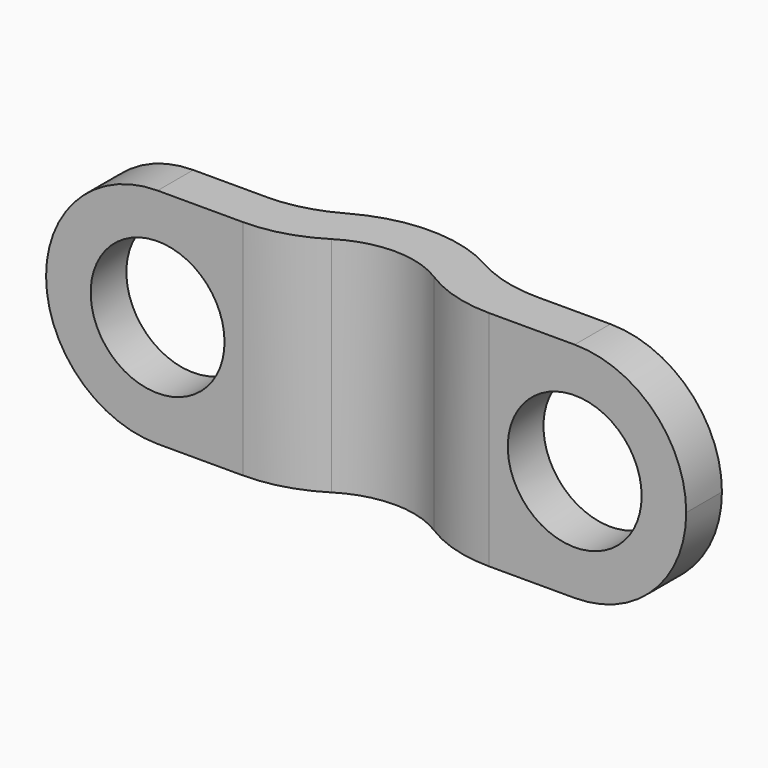
from build123d import *

# Parameters (mm, degrees)
F1_DEPTH      = 2.5
F1_DEPTH_BACK = 2.5
F2_R          = 2.49999
F3_R          = 1.5
F4_DEPTH      = 25
F5_R          = 3


# Not quite as in the source:
# - a fillet or chamfer is up to 0.001 mm smaller than in the source, because OpenCascade refuses the exact size


with BuildPart() as f1:
    # F0 (on Top) → F1 (new body, two sides)
    with BuildSketch(Plane.XY) as f1_sk:
        with BuildLine():
            Line((-6.175, 0), (-4.675, 0))
            Line((-4.675, 0), (-3.175, 0))
            Line((-3.175, 0), (-1.675, 0))
            ThreePointArc((-1.675, 0), (-0.9276877762, 0.5883021777), (0, 0.7979933839))
            Line((0, 0.7979933839), (0, 1))
            Line((0, 1), (-2.0980018512, 1))
            Line((-2.0980018512, 1), (-7.175, 1))
            Line((-7.175, 1), (-7.175, 0))
            Line((-7.175, 0), (-6.175, 0))
        make_face()
        with BuildLine():
            Line((-2.0980018512, 1), (0, 1))
            Line((0, 1), (2.0980018512, 1))
            ThreePointArc((2.0980018512, 1), (0, 1.7979933839), (-2.0980018512, 1))
        make_face()
        with BuildLine():
            Line((0, 1), (0, 0.7979933839))
            ThreePointArc((0, 0.7979933839), (0.9276877762, 0.5883021777), (1.675, 0))
            Line((1.675, 0), (3.175, 0))
            Line((3.175, 0), (4.675, 0))
            Line((4.675, 0), (6.175, 0))
            Line((6.175, 0), (7.175, 0))
            Line((7.175, 0), (7.175, 1))
            Line((7.175, 1), (2.0980018512, 1))
            Line((2.0980018512, 1), (0, 1))
        make_face()
    extrude(amount=F1_DEPTH)
    extrude(f1_sk.sketch, amount=-F1_DEPTH_BACK)

    # F2 (radius 2.5 in the source; OpenCascade refuses exactly that, so slightly less here)
    f2_edges = [f1.edges().sort_by_distance(p)[0] for p in [
        (7.175, 0.5, 2.5),
        (7.175, 0.5, -2.5),
        (-7.175, 0.5, 2.5),
        (-7.175, 0.5, -2.5),
    ]]
    fillet(f2_edges, radius=F2_R)

    # F3 (on face) → F4 (cut)
    with BuildSketch(Plane.XZ):
        with BuildLine():
            ThreePointArc((3.175, 0), (4.675, -1.5), (6.175, 0))
            ThreePointArc((6.175, 0), (4.675, 1.5), (3.175, 0))
        make_face()
        with Locations((-4.675, 0)):
            Circle(F3_R)
    extrude(amount=-F4_DEPTH, mode=Mode.SUBTRACT)

    # F5
    f5_edges = [f1.edges().sort_by_distance(p)[0] for p in [
        (1.675, 0, 0),
        (-1.675, 0, 0),
        (-2.098002, 1, 0),
        (2.098002, 1, 0),
    ]]
    fillet(f5_edges, radius=F5_R)


solid = f1.part
